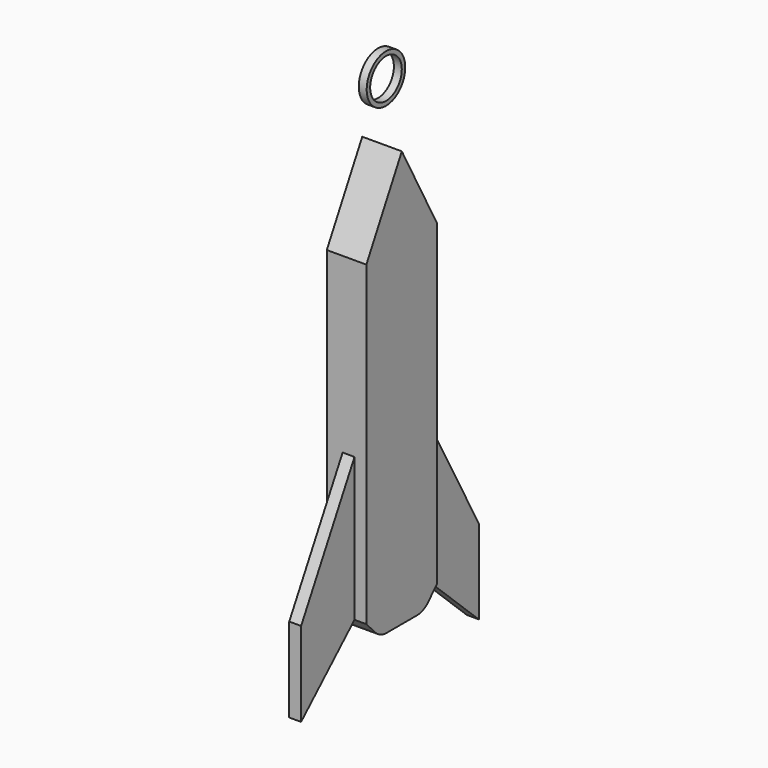
from build123d import *

# Parameters (mm, degrees)
F1_DEPTH = 10
F2_DEPTH = 3
F0_R     = 6.0897341093
F0_R_2   = 4.9929297321
F3_DEPTH = 2


# Not quite as in the source:
# - the program builds the solid bodies; features that only make, move or delete a surface that nothing else refers to are left out


with BuildPart() as f1:
    # F0 (on Right) → F1 (new body)
    with BuildSketch(Plane.YZ):
        Polygon((11.1955845308, 38.1733139123), (0, 58.8363524846), (-11.1955845308, 38.1733139123), (-11.1955845308, -5.587994291), (-11.1955845308, -41.8266860877), (11.1955845308, -41.8266860877), (11.1955845308, -5.587994291), align=None)
        with BuildLine():
            Line((11.1955845308, -41.8266860877), (-11.1955845308, -41.8266860877))
            Line((-11.1955845308, -41.8266860877), (-8.3940999014, -44.8032632523))
            ThreePointArc((-8.3940999014, -44.8032632523), (-6.7362644429, -45.9663262157), (-4.753100084, -46.3764396021))
            Line((-4.753100084, -46.3764396021), (4.753100084, -46.3764396021))
            ThreePointArc((4.753100084, -46.3764396021), (6.7362644429, -45.9663262157), (8.3940999014, -44.8032632523))
            Line((8.3940999014, -44.8032632523), (11.1955845308, -41.8266860877))
        make_face()
    extrude(amount=-F1_DEPTH)


with BuildPart() as f2:
    # F0 (on Right) → F2 (new body)
    with BuildSketch(Plane.YZ):
        Polygon((28.0629971228, -36.3462130386), (11.1955845308, -5.587994291), (11.1955845308, -41.8266860877), (28.0629971228, -57.7018992944), align=None)
    extrude(amount=F2_DEPTH)


with BuildPart() as f2b:
    # F0 (on Right) → F2, piece 2 (new body)
    with BuildSketch(Plane.YZ):
        Polygon((-11.1955845308, -41.8266860877), (-11.1955845308, -5.587994291), (-28.0629971228, -36.3462130386), (-28.0629971228, -57.7018992944), align=None)
    extrude(amount=F2_DEPTH)


with BuildPart() as f3:
    # F0 (on Right) → F3 (new body)
    with BuildSketch(Plane.YZ):
        with Locations((0, 73.7337560306)):
            Circle(F0_R)
        with Locations((0, 73.7337560306)):
            Circle(F0_R_2, mode=Mode.SUBTRACT)
    extrude(amount=F3_DEPTH)


with BuildPart() as f2_1:
    # F5: moved
    add(f2.part.moved(Location((-6, 0, 0))))


with BuildPart() as f2b_1:
    # F6: moved
    add(f2b.part.moved(Location((-6, 0, 0))))


with BuildPart() as f3_1:
    # F7: moved
    add(f3.part.moved(Location((-6, 0, 0))))


solid = Compound([f1.part, f2_1.part, f2b_1.part, f3_1.part])
